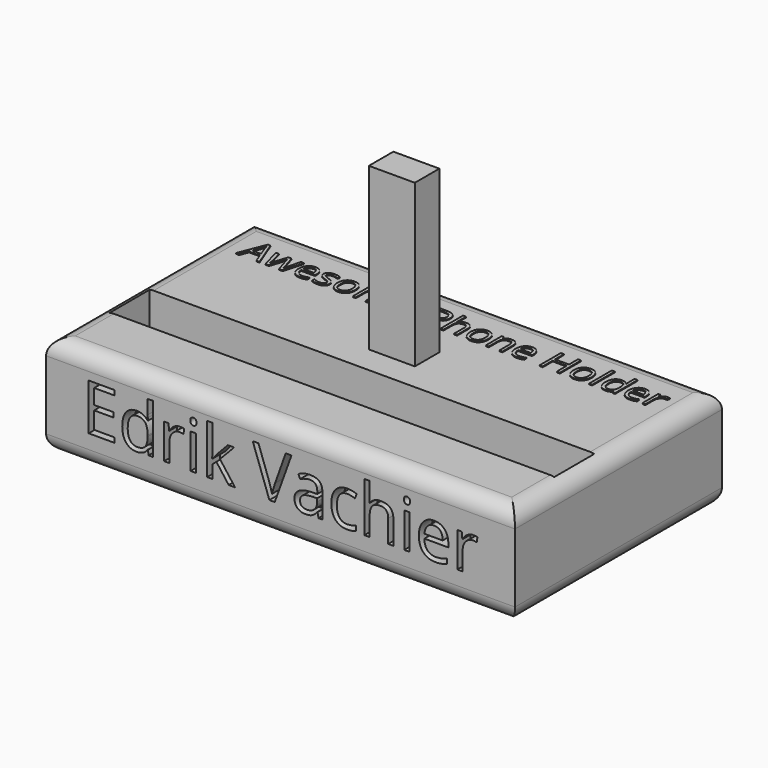
from build123d import *

# Parameters (mm, degrees)
F0_W          = 81.28
F0_H          = 31.75
F1_DEPTH      = 73.66
F1_DEPTH_BACK = 73.66
F3_DEPTH      = 12.7
F4_W          = 7.8205270693
F4_H          = 9.6252644435
F4_W_2        = 6.6173691303
F5_DEPTH      = 50.8
F6_TEXT_SIZE  = 20.4703958136
F7_DEPTH      = 5.08
F8_TEXT_SIZE  = 8.355263142
F9_DEPTH      = 2.54
F10_TEXT_SIZE = 11.697364971
F11_DEPTH     = 0.254
F12_T1_DEPTH  = 172.72
F12_T3_DEPTH  = 106.68


# Not quite as in the source:
# - a fillet or chamfer that OpenCascade refuses, or shapes differently, is made with other operations: its cross-section is extruded or revolved along the edge and cut away or added
# - Text() gives the source's letters only with a copy of the font that has no kerning and outlines rounded to 1/6400 em; it was checked with that copy


with BuildPart() as f1:
    # F0 (on Right) → F1 (new body, two sides)
    with BuildSketch(Plane.YZ) as f1_sk:
        with Locations((10.2995780601, -3.325394626)):
            Rectangle(F0_W, F0_H)
    extrude(amount=F1_DEPTH)
    extrude(f1_sk.sketch, amount=-F1_DEPTH_BACK)

    # F2 (on face) → F3 (cut)
    with BuildSketch(Plane.XY.offset(12.549605374)):
        Polygon((0, 5.55625), (-69.85, 5.55625), (-69.85, 0), (-69.85, -10.16), (0, -10.16), (69.85, -10.16), (69.85, 0), (69.85, 5.55625), align=None)
    extrude(amount=-F3_DEPTH, mode=Mode.SUBTRACT)

    # F4 (on face) → F5 (join)
    with BuildSketch(Plane.XY.offset(12.549605374)):
        with Locations((-3.9102635346, 18.9497373067)):
            Rectangle(F4_W, F4_H)
        with Locations((3.3086845651, 18.9497373067)):
            Rectangle(F4_W_2, F4_H)
    extrude(amount=F5_DEPTH)

    # F6 (on face) → F7 (cut)
    with BuildSketch(Plane.XZ.offset(30.3404219399)):
        with Locations((-62.2634217143, -9.6252639778)):
            Text('Edrik Vachier', F6_TEXT_SIZE, font='Open Sans', text_align=(TextAlign.LEFT, TextAlign.BOTTOM))
    extrude(amount=-F7_DEPTH, mode=Mode.SUBTRACT)

    # F8 (on face) → F9 (cut)
    with BuildSketch(Plane.XY.offset(-0.150394626)):
        with Locations((-65.4112663231, -6.0157894623)):
            Text('The Place Where The Phone Goes', F8_TEXT_SIZE, font='Open Sans', text_align=(TextAlign.LEFT, TextAlign.BOTTOM))
    extrude(amount=-F9_DEPTH, mode=Mode.SUBTRACT)

    # F10 (on face) → F11 (join)
    with BuildSketch(Plane.XY.offset(12.549605374)):
        with Locations((-64.9705305696, 33.3876311779)):
            Text('Awesome Phone Holder', F10_TEXT_SIZE, font='Open Sans', text_align=(TextAlign.LEFT, TextAlign.BOTTOM))
    extrude(amount=F11_DEPTH)

    # F12: fillet of radius 5.08 on 8 edges, made by hand

    # F12_s2 → F12_t1 (cut)
    with BuildSketch(Plane.YZ.offset(-86.36)):
        with BuildLine():
            ThreePointArc((-25.2604219399, 12.549605374), (-28.8525243883, 11.0617078225), (-30.3404219399, 7.469605374))
            Line((-30.3404219399, 7.469605374), (-30.3404219399, 12.549605374))
            Line((-30.3404219399, 12.549605374), (-25.2604219399, 12.549605374))
        make_face()
        with BuildLine():
            ThreePointArc((50.9395780601, 7.469605374), (49.4516805085, 11.0617078225), (45.8595780601, 12.549605374))
            Line((45.8595780601, 12.549605374), (50.9395780601, 12.549605374))
            Line((50.9395780601, 12.549605374), (50.9395780601, 7.469605374))
        make_face()
        with BuildLine():
            ThreePointArc((50.9395780601, -14.120394626), (49.4516805085, -17.7124970744), (45.8595780601, -19.200394626))
            Line((45.8595780601, -19.200394626), (50.9395780601, -19.200394626))
            Line((50.9395780601, -19.200394626), (50.9395780601, -14.120394626))
        make_face()
        with BuildLine():
            ThreePointArc((-25.2604219399, -19.200394626), (-28.8525243883, -17.7124970744), (-30.3404219399, -14.120394626))
            Line((-30.3404219399, -14.120394626), (-30.3404219399, -19.200394626))
            Line((-30.3404219399, -19.200394626), (-25.2604219399, -19.200394626))
        make_face()
    extrude(amount=F12_T1_DEPTH, mode=Mode.SUBTRACT)

    # F12_s4 → F12_t3 (cut)
    with BuildSketch(Plane.XZ.offset(-63.6395780601)):
        with BuildLine():
            ThreePointArc((-68.58, 12.549605374), (-72.1721024484, 11.0617078225), (-73.66, 7.469605374))
            Line((-73.66, 7.469605374), (-73.66, 12.549605374))
            Line((-73.66, 12.549605374), (-68.58, 12.549605374))
        make_face()
        with BuildLine():
            ThreePointArc((73.66, 7.469605374), (72.1721024484, 11.0617078225), (68.58, 12.549605374))
            Line((68.58, 12.549605374), (73.66, 12.549605374))
            Line((73.66, 12.549605374), (73.66, 7.469605374))
        make_face()
        with BuildLine():
            ThreePointArc((68.58, -19.200394626), (72.1721024484, -17.7124970744), (73.66, -14.120394626))
            Line((73.66, -14.120394626), (73.66, -19.200394626))
            Line((73.66, -19.200394626), (68.58, -19.200394626))
        make_face()
        with BuildLine():
            ThreePointArc((-68.58, -19.200394626), (-72.1721024484, -17.7124970744), (-73.66, -14.120394626))
            Line((-73.66, -14.120394626), (-73.66, -19.200394626))
            Line((-73.66, -19.200394626), (-68.58, -19.200394626))
        make_face()
    extrude(amount=F12_T3_DEPTH, mode=Mode.SUBTRACT)


solid = f1.part
